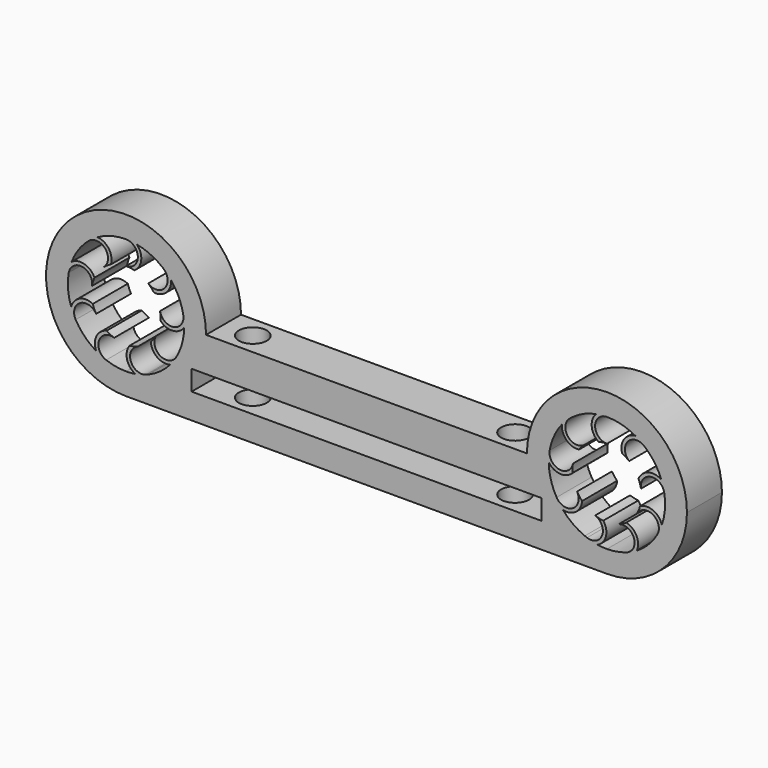
from build123d import *

# Parameters (mm, degrees)
F1_DEPTH = 5
F3_DEPTH = 5
F4_W     = 5
F4_H     = 2.3
F5_DEPTH = 20
F6_R     = 1.6
F7_DEPTH = 18.301


# Not quite as in the source:
# - a pattern or mirror of a feature is missing from the dataset's text; its kind, count and spacing are read off the source's solid


with BuildPart() as f1:
    # F0 (on Front) → F1 (new body)
    with BuildSketch(Plane.XZ):
        with BuildLine():
            ThreePointArc((-27.5, -15.6002467841), (-32.2022600949, -4.2479866892), (-20.85, -8.9502467841))
            Line((-20.85, -8.9502467841), (-18.35, -8.9502467841))
            ThreePointArc((-18.35, -8.9502467841), (-33.9700270479, -2.4802197362), (-27.5, -18.1002467841))
            Line((-27.5, -18.1002467841), (-27.5, -15.6002467841))
        make_face()
        with BuildLine():
            Line((-18.35, -8.9502467841), (-20.85, -8.9502467841))
            Line((-20.85, -8.9502467841), (-20.85, -15.1002467841))
            Line((-20.85, -15.1002467841), (-20.7250461256, -15.1002467841))
            ThreePointArc((-20.7250461256, -15.1002467841), (-18.9643884826, -12.2465835425), (-18.35, -8.9502467841))
        make_face()
        with BuildLine():
            ThreePointArc((-24.9701778719, -15.1002467841), (-26.2106203042, -15.4740493562), (-27.5, -15.6002467841))
            Line((-27.5, -15.6002467841), (-27.5, -18.1002467841))
            ThreePointArc((-27.5, -18.1002467841), (-23.7952732894, -17.3166976445), (-20.7250461256, -15.1002467841))
            Line((-20.7250461256, -15.1002467841), (-20.85, -15.1002467841))
            Line((-20.85, -15.1002467841), (-24.9701778719, -15.1002467841))
        make_face()
        with BuildLine():
            Line((18.35, -8.9502467841), (-18.35, -8.9502467841))
            ThreePointArc((-18.35, -8.9502467841), (-18.9643884826, -12.2465835425), (-20.7250461256, -15.1002467841))
            Line((-20.7250461256, -15.1002467841), (20.7250461256, -15.1002467841))
            ThreePointArc((20.7250461256, -15.1002467841), (18.9643884826, -12.2465835425), (18.35, -8.9502467841))
        make_face()
        with BuildLine():
            ThreePointArc((-20.7250461256, -15.1002467841), (-23.7952732894, -17.3166976445), (-27.5, -18.1002467841))
            Line((-27.5, -18.1002467841), (27.5, -18.1002467841))
            ThreePointArc((27.5, -18.1002467841), (23.7952732894, -17.3166976445), (20.7250461256, -15.1002467841))
            Line((20.7250461256, -15.1002467841), (-20.7250461256, -15.1002467841))
        make_face()
        with BuildLine():
            Line((20.85, -8.9502467841), (18.35, -8.9502467841))
            ThreePointArc((18.35, -8.9502467841), (18.9643884826, -12.2465835425), (20.7250461256, -15.1002467841))
            Line((20.7250461256, -15.1002467841), (20.85, -15.1002467841))
            Line((20.85, -15.1002467841), (20.85, -8.9502467841))
        make_face()
        with BuildLine():
            ThreePointArc((36.65, -8.9502467841), (27.5, 0.1997532159), (18.35, -8.9502467841))
            Line((18.35, -8.9502467841), (20.85, -8.9502467841))
            ThreePointArc((20.85, -8.9502467841), (27.5, -2.3002467841), (34.15, -8.9502467841))
            ThreePointArc((34.15, -8.9502467841), (32.2022600949, -13.652506879), (27.5, -15.6002467841))
            Line((27.5, -15.6002467841), (27.5, -18.1002467841))
            ThreePointArc((27.5, -18.1002467841), (33.9700270479, -15.4202738319), (36.65, -8.9502467841))
        make_face()
        with BuildLine():
            ThreePointArc((20.7250461256, -15.1002467841), (23.7952732894, -17.3166976445), (27.5, -18.1002467841))
            Line((27.5, -18.1002467841), (27.5, -15.6002467841))
            ThreePointArc((27.5, -15.6002467841), (26.2106203042, -15.4740493562), (24.9701778719, -15.1002467841))
            Line((24.9701778719, -15.1002467841), (20.85, -15.1002467841))
            Line((20.85, -15.1002467841), (20.7250461256, -15.1002467841))
        make_face()
        with BuildLine():
            Line((-20.85, -15.1002467841), (-20.85, -8.9502467841))
            ThreePointArc((-20.85, -8.9502467841), (-21.9752458357, -12.6515426955), (-24.9701778719, -15.1002467841))
            Line((-24.9701778719, -15.1002467841), (-20.85, -15.1002467841))
        make_face()
        with BuildLine():
            ThreePointArc((24.9701778719, -15.1002467841), (21.9752458357, -12.6515426955), (20.85, -8.9502467841))
            Line((20.85, -8.9502467841), (20.85, -15.1002467841))
            Line((20.85, -15.1002467841), (24.9701778719, -15.1002467841))
        make_face()
    extrude(amount=F1_DEPTH)

    # F2 (on face) → F3 (join, through all)
    with BuildSketch(Plane(origin=(0, 0, 0), x_dir=(-1, 0, 0), z_dir=(0, 1, 0))):
        with BuildLine():
            ThreePointArc((27.5, -5.0002467841), (26.15, -3.6502467841), (27.5, -2.3002467841))
            ThreePointArc((27.5, -2.3002467841), (26.8763316072, -2.3295566587), (26.2581608513, -2.4172279162))
            ThreePointArc((26.2581608513, -2.4172279162), (25.7598479988, -3.8356409932), (26.5458163918, -5.1172279162))
            ThreePointArc((26.5458163918, -5.1172279162), (27.0193361509, -5.0296011403), (27.5, -5.0002467841))
        make_face()
        with BuildLine():
            ThreePointArc((24.9609889417, -5.9243712338), (23.0590656705, -5.7579745086), (23.2254623956, -3.8560512373))
            ThreePointArc((23.2254623956, -3.8560512373), (22.7665447132, -4.2793902194), (22.3493524387, -4.7439028016))
            ThreePointArc((22.3493524387, -4.7439028016), (22.8793609985, -6.1507795846), (24.3052359132, -6.6273213807))
            ThreePointArc((24.3052359132, -6.6273213807), (24.6116476876, -6.2558227419), (24.9609889417, -5.9243712338))
        make_face()
        with BuildLine():
            ThreePointArc((23.6100093756, -8.2643364823), (22.0460938692, -9.359401909), (20.9510284425, -7.7954864026))
            ThreePointArc((20.9510284425, -7.7954864026), (20.8715941544, -8.4147694774), (20.8505892632, -9.0387727847))
            ThreePointArc((20.8505892632, -9.0387727847), (22.1609223396, -9.7758199912), (23.5595210567, -9.2243374579))
            ThreePointArc((23.5595210567, -9.2243374579), (23.5554513717, -8.742795298), (23.6100093756, -8.2643364823))
        make_face()
        with BuildLine():
            ThreePointArc((21.7409310648, -12.2752467841), (22.0781483573, -12.8007045184), (22.4631592713, -13.2922204683))
            ThreePointArc((22.4631592713, -13.2922204683), (23.9406974553, -13.014565519), (24.6576000913, -11.6931034626))
            ThreePointArc((24.6576000913, -11.6931034626), (24.3449531978, -11.32683671), (24.0791996551, -10.9252467841))
            ThreePointArc((24.0791996551, -10.9252467841), (23.5850653599, -12.7693810792), (21.7409310648, -12.2752467841))
        make_face()
        with BuildLine():
            ThreePointArc((25.2255660469, -15.1992027123), (25.8216472009, -15.3849675925), (26.4325230347, -15.5140104094))
            ThreePointArc((26.4325230347, -15.5140104094), (27.3859097889, -14.3515711409), (27.0856696329, -12.878456344))
            ThreePointArc((27.0856696329, -12.878456344), (26.6107364871, -12.7988452828), (26.1490204339, -12.6620326362))
            ThreePointArc((26.1490204339, -12.6620326362), (26.9558782784, -14.3923448677), (25.2255660469, -15.1992027123))
        make_face()
        with BuildLine():
            ThreePointArc((29.7744339531, -15.1992027123), (30.3504659721, -14.9583532863), (30.9013711338, -14.6645424021))
            ThreePointArc((30.9013711338, -14.6645424021), (30.8845062002, -13.1612370672), (29.7076089581, -12.2257563152))
            ThreePointArc((29.7076089581, -12.2257563152), (29.2926160571, -12.4700518457), (28.8509795661, -12.6620326362))
            ThreePointArc((28.8509795661, -12.6620326362), (30.5812917977, -13.4688904808), (29.7744339531, -15.1992027123))
        make_face()
        with BuildLine():
            ThreePointArc((33.2590689352, -12.2752467841), (33.5455200355, -11.7204791751), (33.7786798774, -11.1412919678))
            ThreePointArc((33.7786798774, -11.1412919678), (32.7994545459, -10.0005338401), (31.2965835169, -10.0404089735))
            ThreePointArc((31.2965835169, -10.0404089735), (31.1357106513, -10.494302502), (30.9208003449, -10.9252467841))
            ThreePointArc((30.9208003449, -10.9252467841), (32.7649346401, -10.431112489), (33.2590689352, -12.2752467841))
        make_face()
        with BuildLine():
            ThreePointArc((31.3899906244, -8.2643364823), (32.4850560511, -6.7004209759), (34.0489715575, -7.7954864026))
            ThreePointArc((34.0489715575, -7.7954864026), (33.9118080859, -7.1863825404), (33.7181245266, -6.5928271413))
            ThreePointArc((33.7181245266, -6.5928271413), (32.2347292126, -6.3483896268), (31.1090944539, -7.3449626276))
            ThreePointArc((31.1090944539, -7.3449626276), (31.2776158253, -7.7960723276), (31.3899906244, -8.2643364823))
        make_face()
        with BuildLine():
            ThreePointArc((30.0390110583, -5.9243712338), (29.8726143331, -4.0224479625), (31.7745376044, -3.8560512373))
            ThreePointArc((31.7745376044, -3.8560512373), (31.2779398735, -3.4776175885), (30.748039603, -3.1474251655))
            ThreePointArc((30.748039603, -3.1474251655), (29.4545714601, -3.9136832939), (29.2328699852, -5.4006465792))
            ThreePointArc((29.2328699852, -5.4006465792), (29.6519325712, -5.6378932086), (30.0390110583, -5.9243712338))
        make_face()
    f3 = extrude(amount=-F3_DEPTH)

    # F3_copies: F3 across plane
    add(f3.mirror(Plane(origin=(0, 0, 0), x_dir=(0, 0, 1), z_dir=(1, 0, 0))))

    # F4 (on Right) → F5 (cut, symmetric)
    with BuildSketch(Plane.YZ):
        with Locations((-2.5, -14.0502467841)):
            Rectangle(F4_W, F4_H)
    extrude(amount=F5_DEPTH, both=True, mode=Mode.SUBTRACT)

    # F6 (on face) → F7 (cut, through all)
    with BuildSketch(Plane(origin=(0, 0, -18.1002467841), x_dir=(1, 0, 0), z_dir=(0, 0, -1))):
        with Locations((-15, 2.5)):
            Circle(F6_R)
        with Locations((15, 2.5)):
            Circle(F6_R)
    extrude(amount=-F7_DEPTH, mode=Mode.SUBTRACT)


solid = f1.part
